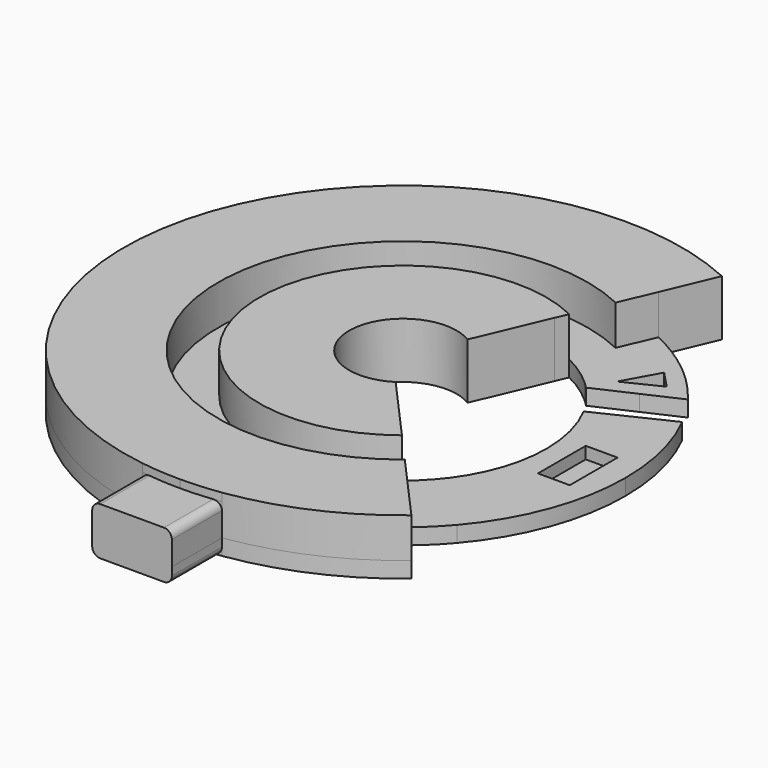
from build123d import *

# Parameters (mm, degrees)
F1_DEPTH     = 4
F2_DEPTH     = 10
F3_W         = 8
F3_H         = 15
F4_DEPTH     = 3
F5_DEPTH     = 4
F6_DEPTH     = 8
F7_T4_DEPTH  = 25.7179676972
F7_S5_R      = 70
F7_T6_DEPTH  = 14
F7_T10_DEPTH = 25.7179676972
F7_S11_R     = 70
F7_T12_DEPTH = 14
F7_T16_DEPTH = 25.7179676972
F7_S17_R     = 70
F7_T18_DEPTH = 14
F7_T22_DEPTH = 25.7179676972
F7_S23_R     = 70
F7_T24_DEPTH = 14


# Not quite as in the source:
# - a fillet or chamfer that OpenCascade refuses, or shapes differently, is made with other operations: its cross-section is extruded or revolved along the edge and cut away or added


with BuildPart() as f1:
    # F0 (on Top) → F1 (new body)
    with BuildSketch(Plane.XY):
        with BuildLine():
            Line((23.5981723771, 50.6307036507), (29.1379201291, 63.6473221004))
            ThreePointArc((29.1379201291, 63.6473221004), (-67.1499688178, 19.7707280537), (-10, -69.2820323028))
            ThreePointArc((-10, -69.2820323028), (-5.0128703757, -69.8202773598), (0, -70))
            ThreePointArc((0, -70), (5.0128703757, -69.8202773598), (10, -69.2820323028))
            ThreePointArc((10, -69.2820323028), (28.5954871466, -63.89286435), (45.0035054679, -53.6160842994))
            Line((45.0035054679, -53.6160842994), (35.576841855, -43.0654178585))
            ThreePointArc((35.576841855, -43.0654178585), (-55.4090369327, -7.0838208542), (23.5981723771, 50.6307036507))
        make_face()
        with BuildLine():
            Line((19.8677907274, 41.8655113026), (23.5981723771, 50.6307036507))
            ThreePointArc((23.5981723771, 50.6307036507), (-55.4090369327, -7.0838208542), (35.576841855, -43.0654178585))
            Line((35.576841855, -43.0654178585), (29.2286049616, -35.9602391123))
            ThreePointArc((29.2286049616, -35.9602391123), (-46.0089760191, -5.5339200114), (19.8677907274, 41.8655113026))
        make_face()
        with BuildLine():
            Line((14.5657325798, 29.407386674), (15.8289323737, 32.3754983065))
            ThreePointArc((15.8289323737, 32.3754983065), (-35.8310083049, -3.8557534328), (22.3545915501, -28.266592071))
            Line((22.3545915501, -28.266592071), (20.2043653008, -25.8599802663))
            ThreePointArc((20.2043653008, -25.8599802663), (-32.6475173449, -3.3308509117), (14.5657325798, 29.407386674))
        make_face()
        with BuildLine():
            Line((6.9658582886, 11.5501360659), (14.5657325798, 29.407386674))
            ThreePointArc((14.5657325798, 29.407386674), (-32.6475173449, -3.3308509117), (20.2043653008, -25.8599802663))
            Line((20.2043653008, -25.8599802663), (7.257370403, -11.3692303905))
            ThreePointArc((7.257370403, -11.3692303905), (-13.4870085006, -0.1715416686), (6.9658582886, 11.5501360659))
        make_face()
        with BuildLine():
            Line((15.8289323737, 32.3754983065), (19.8677907274, 41.8655113026))
            ThreePointArc((19.8677907274, 41.8655113026), (-46.0089760191, -5.5339200114), (29.2286049616, -35.9602391123))
            Line((29.2286049616, -35.9602391123), (22.3545915501, -28.266592071))
            ThreePointArc((22.3545915501, -28.266592071), (-35.8310083049, -3.8557534328), (15.8289323737, 32.3754983065))
        make_face()
        with BuildLine():
            ThreePointArc((32.4763517935, 45.4491855361), (28.1567060881, 48.2446037809), (23.5981723771, 50.6307036507))
            Line((23.5981723771, 50.6307036507), (19.8677907274, 41.8655113026))
            ThreePointArc((19.8677907274, 41.8655113026), (24.3303762174, 39.4396112828), (28.5006543682, 36.5398802079))
            Line((28.5006543682, 36.5398802079), (32.4763517935, 45.4491855361))
        make_face()
        with BuildLine():
            ThreePointArc((28.5006543682, 36.5398802079), (24.3303762174, 39.4396112828), (19.8677907274, 41.8655113026))
            Line((19.8677907274, 41.8655113026), (15.8289323737, 32.3754983065))
            ThreePointArc((15.8289323737, 32.3754983065), (20.1791178088, 29.8585196408), (24.1368343884, 26.7608149426))
            Line((24.1368343884, 26.7608149426), (28.5006543682, 36.5398802079))
        make_face()
        with BuildLine():
            ThreePointArc((35.6941134, 29.5530102292), (32.2869345127, 33.2416005149), (28.5006543682, 36.5398802079))
            Line((28.5006543682, 36.5398802079), (24.1368343884, 26.7608149426))
            ThreePointArc((24.1368343884, 26.7608149426), (25.022522536, 25.9345591175), (25.8799433339, 25.0790056366))
            Line((25.8799433339, 25.0790056366), (35.6941134, 29.5530102292))
        make_face()
        with BuildLine():
            ThreePointArc((44.6112733376, 33.6180930885), (38.9951173125, 39.9965338185), (32.4763517935, 45.4491855361))
            Line((32.4763517935, 45.4491855361), (28.5006543682, 36.5398802079))
            ThreePointArc((28.5006543682, 36.5398802079), (32.2869345127, 33.2416005149), (35.6941134, 29.5530102292))
            Line((35.6941134, 29.5530102292), (44.6112733376, 33.6180930885))
        make_face()
        with BuildLine():
            Line((22.3545915501, -28.266592071), (29.2286049616, -35.9602391123))
            ThreePointArc((29.2286049616, -35.9602391123), (32.8206282453, -32.7147750505), (36.0544716862, -29.1122863487))
            Line((36.0544716862, -29.1122863487), (29.0097989093, -21.3812899032))
            ThreePointArc((29.0097989093, -21.3812899032), (25.9119084265, -25.0459775688), (22.3545915501, -28.266592071))
        make_face()
        with BuildLine():
            Line((29.2286049616, -35.9602391123), (35.576841855, -43.0654178585))
            ThreePointArc((35.576841855, -43.0654178585), (39.2024865114, -39.7933027409), (42.5284655631, -36.2170057923))
            Line((42.5284655631, -36.2170057923), (36.0544716862, -29.1122863487))
            ThreePointArc((36.0544716862, -29.1122863487), (32.8206282453, -32.7147750505), (29.2286049616, -35.9602391123))
        make_face()
        with BuildLine():
            Line((36.0544716862, -29.1122863487), (42.5284655631, -36.2170057923))
            ThreePointArc((42.5284655631, -36.2170057923), (52.4212879012, -19.2963848035), (55.860020513, 0))
            ThreePointArc((55.860020513, 0), (54.3029220862, 13.0971197067), (49.7184350628, 25.4640748234))
            Line((49.7184350628, 25.4640748234), (41.1278773135, 21.3529354587))
            ThreePointArc((41.1278773135, 21.3529354587), (45.0185527566, 10.9899978491), (46.3405885269, 0))
            ThreePointArc((46.3405885269, 0), (43.6934524957, -15.4380165186), (36.0544716862, -29.1122863487))
        make_face()
        with BuildLine():
            Line((29.0097989093, -21.3812899032), (36.0544716862, -29.1122863487))
            ThreePointArc((36.0544716862, -29.1122863487), (43.6934524957, -15.4380165186), (46.3405885269, 0))
            ThreePointArc((46.3405885269, 0), (45.0185527566, 10.9899978491), (41.1278773135, 21.3529354587))
            Line((41.1278773135, 21.3529354587), (31.8282165391, 16.9024442795))
            ThreePointArc((31.8282165391, 16.9024442795), (34.9696231307, 8.7093885424), (36.0378688421, 0))
            ThreePointArc((36.0378688421, 0), (34.2357950026, -11.253369772), (29.0097989093, -21.3812899032))
        make_face()
    extrude(amount=-F1_DEPTH)

    # F0 (on Top) → F2 (join)
    with BuildSketch(Plane.XY):
        with BuildLine():
            Line((23.5981723771, 50.6307036507), (29.1379201291, 63.6473221004))
            ThreePointArc((29.1379201291, 63.6473221004), (-67.1499688178, 19.7707280537), (-10, -69.2820323028))
            ThreePointArc((-10, -69.2820323028), (-5.0128703757, -69.8202773598), (0, -70))
            ThreePointArc((0, -70), (5.0128703757, -69.8202773598), (10, -69.2820323028))
            ThreePointArc((10, -69.2820323028), (28.5954871466, -63.89286435), (45.0035054679, -53.6160842994))
            Line((45.0035054679, -53.6160842994), (35.576841855, -43.0654178585))
            ThreePointArc((35.576841855, -43.0654178585), (-55.4090369327, -7.0838208542), (23.5981723771, 50.6307036507))
        make_face()
        with BuildLine():
            Line((19.8677907274, 41.8655113026), (23.5981723771, 50.6307036507))
            ThreePointArc((23.5981723771, 50.6307036507), (-55.4090369327, -7.0838208542), (35.576841855, -43.0654178585))
            Line((35.576841855, -43.0654178585), (29.2286049616, -35.9602391123))
            ThreePointArc((29.2286049616, -35.9602391123), (-46.0089760191, -5.5339200114), (19.8677907274, 41.8655113026))
        make_face()
        with BuildLine():
            Line((6.9658582886, 11.5501360659), (14.5657325798, 29.407386674))
            ThreePointArc((14.5657325798, 29.407386674), (-32.6475173449, -3.3308509117), (20.2043653008, -25.8599802663))
            Line((20.2043653008, -25.8599802663), (7.257370403, -11.3692303905))
            ThreePointArc((7.257370403, -11.3692303905), (-13.4870085006, -0.1715416686), (6.9658582886, 11.5501360659))
        make_face()
        with BuildLine():
            Line((14.5657325798, 29.407386674), (15.8289323737, 32.3754983065))
            ThreePointArc((15.8289323737, 32.3754983065), (-35.8310083049, -3.8557534328), (22.3545915501, -28.266592071))
            Line((22.3545915501, -28.266592071), (20.2043653008, -25.8599802663))
            ThreePointArc((20.2043653008, -25.8599802663), (-32.6475173449, -3.3308509117), (14.5657325798, 29.407386674))
        make_face()
    extrude(amount=F2_DEPTH)

    # F3 (on face) → F4 (cut)
    with BuildSketch(Plane.XY):
        Polygon((37.9851715346, 35.276671204), (33.8525412993, 39.626541011), (29.0030042003, 30.8811427968), align=None)
        with Locations((45.2681102753, -1.745258756)):
            Rectangle(F3_W, F3_H)
    extrude(amount=-F4_DEPTH, mode=Mode.SUBTRACT)

    # F0 (on Top) → F5 (join)
    with BuildSketch(Plane.XY):
        with BuildLine():
            ThreePointArc((0, -70), (-5.0128703757, -69.8202773598), (-10, -69.2820323028))
            Line((-10, -69.2820323028), (-10, -74.2803270693))
            ThreePointArc((-10, -74.2803270693), (-5.0112133817, -74.7827167864), (0, -74.9504302157))
            Line((0, -74.9504302157), (0, -70))
        make_face()
        with BuildLine():
            ThreePointArc((10, -69.2820323028), (5.0128703757, -69.8202773598), (0, -70))
            Line((0, -70), (0, -74.9504302157))
            ThreePointArc((0, -74.9504302157), (5.0112133817, -74.7827167864), (10, -74.2803270693))
            Line((10, -74.2803270693), (10, -69.2820323028))
        make_face()
        with BuildLine():
            ThreePointArc((10, -74.2803270693), (5.0112133817, -74.7827167864), (0, -74.9504302157))
            Line((0, -74.9504302157), (0, -85))
            Line((0, -85), (10, -85))
            Line((10, -85), (10, -74.2803270693))
        make_face()
        with BuildLine():
            ThreePointArc((0, -74.9504302157), (-5.0112133817, -74.7827167864), (-10, -74.2803270693))
            Line((-10, -74.2803270693), (-10, -85))
            Line((-10, -85), (0, -85))
            Line((0, -85), (0, -74.9504302157))
        make_face()
    extrude(amount=-F5_DEPTH)

    # F0 (on Top) → F6 (join)
    with BuildSketch(Plane.XY):
        with BuildLine():
            ThreePointArc((0, -70), (-5.0128703757, -69.8202773598), (-10, -69.2820323028))
            Line((-10, -69.2820323028), (-10, -74.2803270693))
            ThreePointArc((-10, -74.2803270693), (-5.0112133817, -74.7827167864), (0, -74.9504302157))
            Line((0, -74.9504302157), (0, -70))
        make_face()
        with BuildLine():
            ThreePointArc((0, -74.9504302157), (-5.0112133817, -74.7827167864), (-10, -74.2803270693))
            Line((-10, -74.2803270693), (-10, -85))
            Line((-10, -85), (0, -85))
            Line((0, -85), (0, -74.9504302157))
        make_face()
        with BuildLine():
            ThreePointArc((10, -69.2820323028), (5.0128703757, -69.8202773598), (0, -70))
            Line((0, -70), (0, -74.9504302157))
            ThreePointArc((0, -74.9504302157), (5.0112133817, -74.7827167864), (10, -74.2803270693))
            Line((10, -74.2803270693), (10, -69.2820323028))
        make_face()
        with BuildLine():
            ThreePointArc((10, -74.2803270693), (5.0112133817, -74.7827167864), (0, -74.9504302157))
            Line((0, -74.9504302157), (0, -85))
            Line((0, -85), (10, -85))
            Line((10, -85), (10, -74.2803270693))
        make_face()
    extrude(amount=F6_DEPTH)

    # F7: fillet of radius 2 on 4 edges, made by hand


with BuildPart() as f7_tool2:
    # F7_s3 → F7_t4 (new body)
    with BuildSketch(Plane.XZ.offset(90)):
        with BuildLine():
            ThreePointArc((10, 6), (9.4142135624, 7.4142135624), (8, 8))
            Line((8, 8), (10, 8))
            Line((10, 8), (10, 6))
        make_face()
    extrude(amount=-F7_T4_DEPTH)

    # F7_s5 → F7_t6 (cut, symmetric)
    with BuildSketch(Plane.XY.offset(7)):
        Circle(F7_S5_R)
    extrude(amount=F7_T6_DEPTH, both=True, mode=Mode.SUBTRACT)


with BuildPart() as f1_1:
    add(f1.part)

    # F7_t1: cut F7_tool2
    add(f7_tool2.part, mode=Mode.SUBTRACT)


with BuildPart() as f7_tool8:
    # F7_s9 → F7_t10 (new body)
    with BuildSketch(Plane.XZ.offset(64.2820323028)):
        with BuildLine():
            ThreePointArc((-8, 8), (-9.4142135624, 7.4142135624), (-10, 6))
            Line((-10, 6), (-10, 8))
            Line((-10, 8), (-8, 8))
        make_face()
    extrude(amount=F7_T10_DEPTH)

    # F7_s11 → F7_t12 (cut, symmetric)
    with BuildSketch(Plane.XY.offset(7)):
        Circle(F7_S11_R)
    extrude(amount=F7_T12_DEPTH, both=True, mode=Mode.SUBTRACT)


with BuildPart() as f1_2:
    add(f1_1.part)

    # F7_t7: cut F7_tool8
    add(f7_tool8.part, mode=Mode.SUBTRACT)


with BuildPart() as f7_tool14:
    # F7_s15 → F7_t16 (new body)
    with BuildSketch(Plane.XZ.offset(90)):
        with BuildLine():
            ThreePointArc((10, -2), (9.4142135624, -3.4142135624), (8, -4))
            Line((8, -4), (10, -4))
            Line((10, -4), (10, -2))
        make_face()
    extrude(amount=-F7_T16_DEPTH)

    # F7_s17 → F7_t18 (cut, symmetric)
    with BuildSketch(Plane.XY.offset(-3)):
        Circle(F7_S17_R)
    extrude(amount=F7_T18_DEPTH, both=True, mode=Mode.SUBTRACT)


with BuildPart() as f1_3:
    add(f1_2.part)

    # F7_t13: cut F7_tool14
    add(f7_tool14.part, mode=Mode.SUBTRACT)


with BuildPart() as f7_tool20:
    # F7_s21 → F7_t22 (new body)
    with BuildSketch(Plane.XZ.offset(64.2820323028)):
        with BuildLine():
            ThreePointArc((-10, -2), (-9.4142135624, -3.4142135624), (-8, -4))
            Line((-8, -4), (-10, -4))
            Line((-10, -4), (-10, -2))
        make_face()
    extrude(amount=F7_T22_DEPTH)

    # F7_s23 → F7_t24 (cut, symmetric)
    with BuildSketch(Plane.XY.offset(-3)):
        Circle(F7_S23_R)
    extrude(amount=F7_T24_DEPTH, both=True, mode=Mode.SUBTRACT)


with BuildPart() as f1_4:
    add(f1_3.part)

    # F7_t19: cut F7_tool20
    add(f7_tool20.part, mode=Mode.SUBTRACT)


solid = f1_4.part
